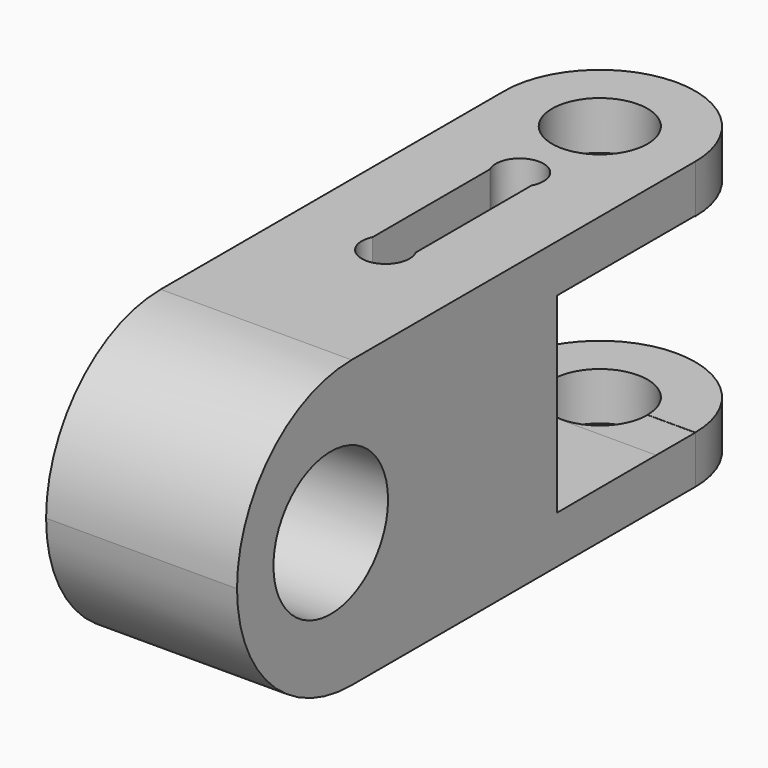
from build123d import *

# Parameters (mm, degrees)
F0_R      = 12.7
F1_DEPTH  = 76.2
F2_R      = 38.09999
F3_R      = 19.05
F4_DEPTH  = 50.801
F6_DEPTH  = 76.201
F8_DEPTH  = 50.801
F11_DEPTH = 50.801


# Not quite as in the source:
# - a fillet or chamfer is up to 0.001 mm smaller than in the source, because OpenCascade refuses the exact size


with BuildPart() as f1:
    # F0 (on Top) → F1 (new body)
    with BuildSketch(Plane.XY):
        with BuildLine():
            Line((25.4, -152.4), (25.4, 0))
            ThreePointArc((25.4, 0), (0, 25.4), (-25.4, 0))
            Line((-25.4, 0), (-25.4, -152.4))
            Line((-25.4, -152.4), (25.4, -152.4))
        make_face()
        Circle(F0_R, mode=Mode.SUBTRACT)
    extrude(amount=F1_DEPTH)

    # F2 (radius 38.1 in the source; OpenCascade refuses exactly that, so slightly less here)
    f2_edges = [f1.edges().sort_by_distance(p)[0] for p in [
        (0, -152.4, 76.2),
        (0, -152.4, 0),
    ]]
    fillet(f2_edges, radius=F2_R)

    # F3 (on face) → F4 (cut, through all)
    with BuildSketch(Plane.YZ.offset(25.4)):
        with Locations((-121.2292984128, 38.5233350098)):
            Circle(F3_R)
    extrude(amount=-F4_DEPTH, mode=Mode.SUBTRACT)

    # F5 (on face) → F6 (cut, through all)
    with BuildSketch(Plane.XY.offset(76.2)):
        with BuildLine():
            Line((-5.7387360482, -29.3549266663), (-5.6882195357, -68.4034783226))
            ThreePointArc((-5.6882195357, -68.4034783226), (0.0700403354, -77.5756190124), (5.6245744634, -68.2786909069))
            Line((5.6245744634, -68.2786909069), (5.5746364254, -29.6772918832))
            ThreePointArc((5.5746364254, -29.6772918832), (0.1808646036, -20.2891562763), (-5.7387360482, -29.3549266663))
        make_face()
    extrude(amount=-F6_DEPTH, mode=Mode.SUBTRACT)

    # F7 (on face) → F8 (cut, through all)
    with BuildSketch(Plane(origin=(-25.4, 0, 0), x_dir=(0, -1, 0), z_dir=(-1, 0, 0))):
        Polygon((0, 63.5), (0, 12.7), (12.9918251187, 12.7), (46.0542105138, 12.633157894), (46.0542105138, 63.5), (12.9918251187, 63.5), align=None)
    extrude(amount=-F8_DEPTH, mode=Mode.SUBTRACT)

    # F10 (on offset) → F11 (cut, through all)
    with BuildSketch(Plane.YZ.offset(25.4)):
        Polygon((25.4299268126, 63.3701309562), (0, 63.3701309562), (0, 12.7395335585), (25.4423227161, 12.7395335585), align=None)
    extrude(amount=-F11_DEPTH, mode=Mode.SUBTRACT)


solid = f1.part
